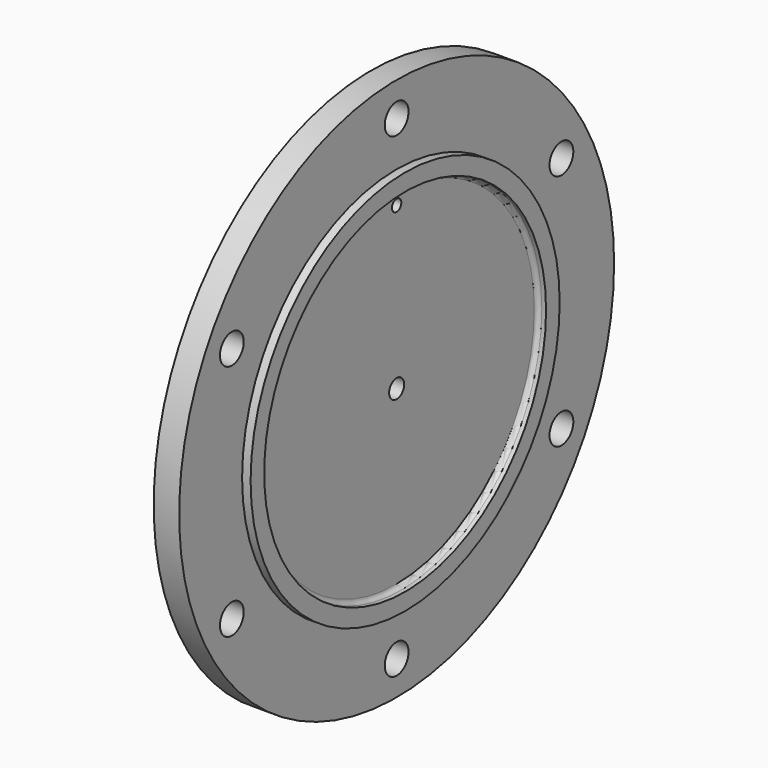
from build123d import *

# Parameters (mm, degrees)
F0_R           = 203.2
F1_DEPTH       = 19.05
F2_R           = 144.399
F2_R_2         = 131.699
F3_DEPTH       = 6.35
F4_R           = 3.175
F6_D           = 22.225
F8_D           = 14
F8_CBORE_D     = 24
F8_CBORE_DEPTH = 7.5
F9_W           = 12.7
F9_H           = 38.1
F10_DEPTH      = 45.72
F12_D          = 5.1054
F12_DEPTH      = 15.875
F12_TIP        = 1.5338169022
F14_D          = 8.73125


# Not quite as in the source:
# - a length typed as a fraction of an inch, garbled in the dataset ("3 / 203.2 mm" for 3/8 in), is restored


with BuildPart() as f1:
    # F0 (on Right) → F1 (new body)
    with BuildSketch(Plane.YZ):
        Circle(F0_R)
    extrude(amount=-F1_DEPTH)

    # F2 (on face) → F3 (join)
    with BuildSketch(Plane.YZ):
        Circle(F2_R)
        Circle(F2_R_2, mode=Mode.SUBTRACT)
    extrude(amount=F3_DEPTH)

    # F4
    f4_edges = [f1.edges().sort_by_distance(p)[0] for p in [
        (0, -131.699, 0),
    ]]
    fillet(f4_edges, radius=F4_R)

    # F6 (through all)
    with Locations(Plane(origin=(-19.05, 0, 0), x_dir=(0, -1, 0), z_dir=(-1, 0, 0))):
        with Locations((0, 177.8), (153.9793167929, 88.9), (-153.9793167929, 88.9), (-153.9793167929, -88.9), (153.9793167929, -88.9), (0, -177.8)):
            Hole(F6_D / 2)

    # F8 (through all)
    with Locations(Plane(origin=(-19.05, 0, 0), x_dir=(0, -1, 0), z_dir=(-1, 0, 0))):
        with Locations((0, 0)):
            CounterBoreHole(F8_D / 2, F8_CBORE_D / 2, F8_CBORE_DEPTH)

    # F9 (on face) → F10 (join)
    with BuildSketch(Plane(origin=(-19.05, 0, 0), x_dir=(0, -1, 0), z_dir=(-1, 0, 0))):
        with Locations((38.1, 0)):
            Rectangle(F9_W, F9_H)
        with Locations((-38.1, 0)):
            Rectangle(F9_W, F9_H)
    extrude(amount=F10_DEPTH)

    # F12
    with Locations(Plane(origin=(-64.77, 0, 0), x_dir=(0, -1, 0), z_dir=(-1, 0, 0))):
        with Locations((-38.1, 12.7), (-38.1, -12.7), (38.1, 12.7), (38.1, -12.7)):
            Hole(F12_D / 2, depth=F12_DEPTH)
            with Locations((0, 0, -(F12_DEPTH + F12_TIP / 2))):  # 118° drill point
                Cone(0, F12_D / 2, F12_TIP, mode=Mode.SUBTRACT)

    # F14 (through all)
    with Locations(Plane(origin=(-19.05, 0, 0), x_dir=(0, -1, 0), z_dir=(-1, 0, 0))):
        with Locations((0, 120.65)):
            Hole(F14_D / 2)


solid = f1.part
